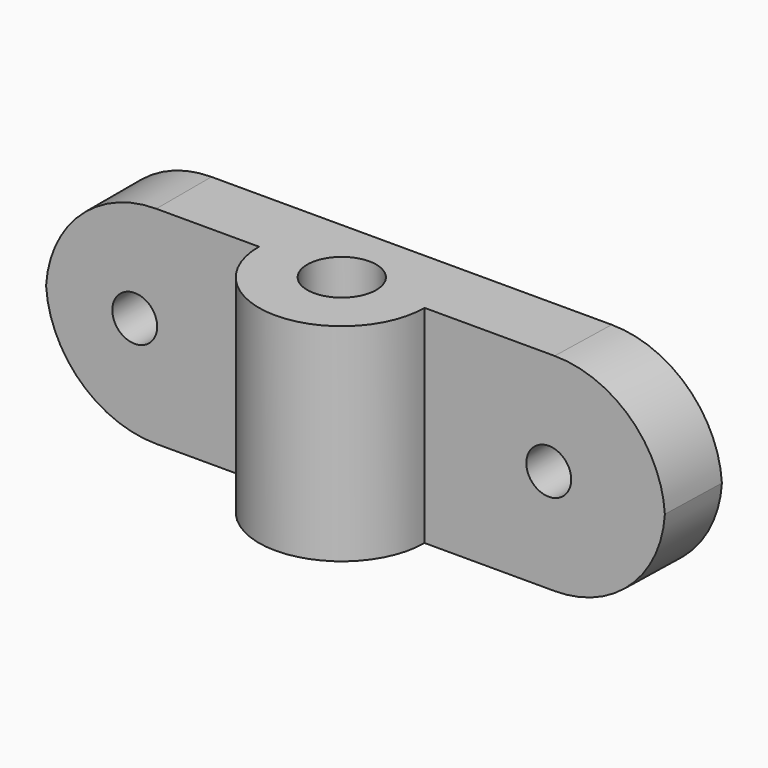
from build123d import *

# Parameters (mm, degrees)
F0_R        = 2.5
F1_DEPTH    = 15
F3_D        = 3.25
F4_T1_DEPTH = 45
F4_T3_DEPTH = 45.0017535366


# Not quite as in the source:
# - a fillet or chamfer that OpenCascade refuses, or shapes differently, is made with other operations: its cross-section is extruded or revolved along the edge and cut away or added


with BuildPart() as f1:
    # F0 (on Top) → F1 (new body)
    with BuildSketch(Plane.XY):
        with BuildLine():
            Line((6, 0), (23.4290786547, 0))
            Line((23.4290786547, 0), (23.5615114343, 5))
            Line((23.5615114343, 5), (-21.4384885657, 5))
            Line((-21.4384885657, 5), (-21.4384885657, 0))
            Line((-21.4384885657, 0), (-6, 0))
            ThreePointArc((-6, 0), (0, -6), (6, 0))
        make_face()
        Circle(F0_R, mode=Mode.SUBTRACT)
    extrude(amount=F1_DEPTH)

    # F3 (through all)
    with Locations(Plane.XZ):
        with Locations((-15, 7.5), (15, 7.5)):
            Hole(F3_D / 2)

    # F4: fillet of radius 8 on 4 edges, made by hand

    # F4_s2 → F4_t1 (cut)
    with BuildSketch(Plane.XZ.offset(-25)):
        with BuildLine():
            ThreePointArc((-13.4384885657, 15), (-19.0953428152, 12.6568542495), (-21.4384885657, 7))
            Line((-21.4384885657, 7), (-21.4384885657, 15))
            Line((-21.4384885657, 15), (-13.4384885657, 15))
        make_face()
        with BuildLine():
            ThreePointArc((-13.4384885657, 0), (-19.0953428152, 2.3431457505), (-21.4384885657, 8))
            Line((-21.4384885657, 8), (-21.4384885657, 0))
            Line((-21.4384885657, 0), (-13.4384885657, 0))
        make_face()
    extrude(amount=F4_T1_DEPTH, mode=Mode.SUBTRACT)

    # F4_s4 → F4_t3 (cut)
    with BuildSketch(Plane(origin=(-0.5131205452, -19.3728677482, 0), x_dir=(0, 0, 1), z_dir=(0.0264772702, 0.9996494156, 0))):
        with BuildLine():
            ThreePointArc((15, 15.4208647858), (12.6568542495, 21.0777190353), (7, 23.4208647858))
            Line((7, 23.4208647858), (15, 23.4208647858))
            Line((15, 23.4208647858), (15, 15.4208647858))
        make_face()
        with BuildLine():
            ThreePointArc((0, 15.4208647858), (2.3431457505, 21.0777190353), (8, 23.4208647858))
            Line((8, 23.4208647858), (0, 23.4208647858))
            Line((0, 23.4208647858), (0, 15.4208647858))
        make_face()
    extrude(amount=F4_T3_DEPTH, mode=Mode.SUBTRACT)


solid = f1.part
